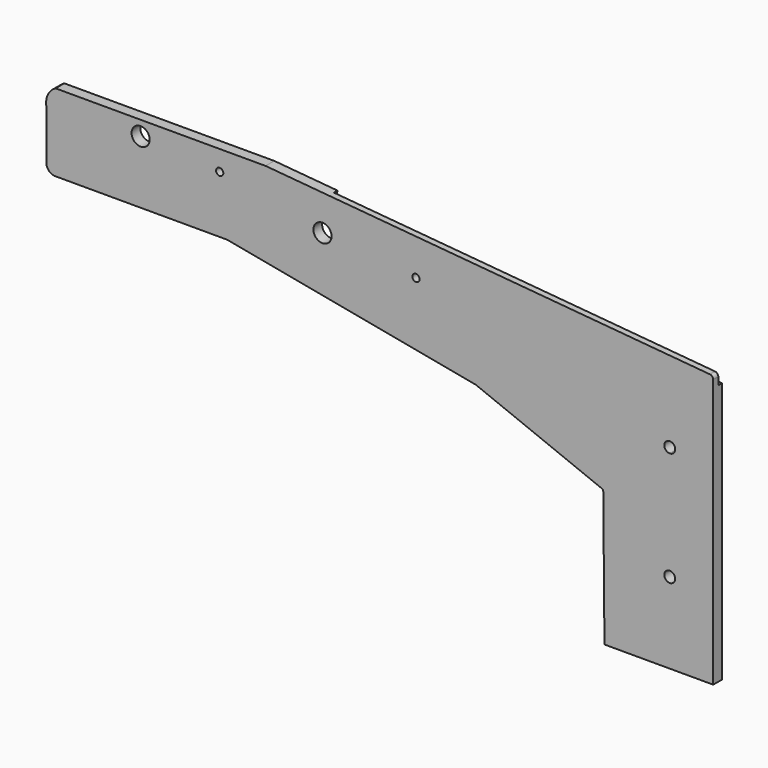
from build123d import *

# Parameters (mm, degrees)
F0_R      = 2
F1_DEPTH  = 6
F3_DEPTH  = 6.001
F5_DEPTH  = 6.001
F6_R      = 5
F7_DEPTH  = 6.001
F8_DEPTH  = 585
F9_R      = 2
F10_DEPTH = 6.001
F12_DEPTH = 2.5
F13_R     = 2


# Not quite as in the source:
# - an extrude ends at something that could not be found from the text; its depth is read off the source's solid


with BuildPart() as f1:
    # F0 (on Front) → F1 (new body)
    with BuildSketch(Plane.XZ):
        with BuildLine():
            Line((61.1081310213, 8.0650188029), (-54.7722764313, 8.0650188029))
            ThreePointArc((-54.7722764313, 8.0650188029), (-58.9525619371, 3.7295520634), (-59.8848706484, -2.2203940898))
            Line((-59.8848706484, -2.2203940898), (-59.8848706484, -29.6689261496))
            ThreePointArc((-59.8848706484, -29.6689261496), (-58.4204045543, -33.2044600555), (-54.8848706484, -34.6689261496))
            Line((-54.8848706484, -34.6689261496), (-38.6363018323, -34.6689261496))
            Line((-38.6363018323, -34.6689261496), (39.8797094822, -34.6689261496))
            Line((39.8797094822, -34.6689261496), (177.1196573973, -60.5151057243))
            Line((177.1196573973, -60.5151057243), (247.381187493, -88.5924363301))
            Line((247.381187493, -88.5924363301), (248.0585300922, -163.5853774846))
            Line((248.0585300922, -163.5853774846), (308.0585300922, -163.5853774846))
            Line((308.0585300922, -163.5853774846), (308.0585300922, -13.5853774846))
            Line((308.0585300922, -13.5853774846), (61.1081310213, 8.0650188029))
        make_face()
        with Locations((35.7915443742, -3.0683759738)):
            Circle(F0_R, mode=Mode.SUBTRACT)
    extrude(amount=F1_DEPTH)

    # F2 (on face) → F3 (cut, through all)
    with BuildSketch(Plane.XZ.offset(6)):
        with BuildLine():
            ThreePointArc((92.5020176823, -9.2679053605), (88.9664837764, -17.8034392664), (97.5020176823, -14.2679053605))
            ThreePointArc((97.5020176823, -14.2679053605), (96.0375515883, -10.7323714546), (92.5020176823, -9.2679053605))
        make_face()
    extrude(amount=-F3_DEPTH, mode=Mode.SUBTRACT)

    # F4 (on face) → F5 (cut, through all)
    with BuildSketch(Plane.XZ.offset(6)):
        with BuildLine():
            ThreePointArc((284.0794362254, -115.9942394993), (281.9581158818, -121.1155598429), (287.0794362254, -118.9942394993))
            ThreePointArc((287.0794362254, -118.9942394993), (286.2007565689, -116.8729191558), (284.0794362254, -115.9942394993))
        make_face()
        with BuildLine():
            ThreePointArc((287.0794362254, -56.0820794532), (281.9581158818, -53.9607591097), (284.0794362254, -59.0820794532))
            ThreePointArc((284.0794362254, -59.0820794532), (286.2007565689, -58.2033997968), (287.0794362254, -56.0820794532))
        make_face()
    extrude(amount=-F5_DEPTH, mode=Mode.SUBTRACT)

    # F6 (on face) → F7 (cut, through all)
    with BuildSketch(Plane(origin=(0, 0, 0), x_dir=(-1, 0, 0), z_dir=(0, 1, 0))):
        with Locations((7.8367077125, 0)):
            Circle(F6_R)
    extrude(amount=-F7_DEPTH, mode=Mode.SUBTRACT)

    # F0 (on Front) → F8 (cut, through all)
    with BuildSketch(Plane.XZ):
        with BuildLine():
            Line((61.1081310213, 8.0650188029), (-54.7722764313, 8.0650188029))
            ThreePointArc((-54.7722764313, 8.0650188029), (-58.9525619371, 3.7295520634), (-59.8848706484, -2.2203940898))
            Line((-59.8848706484, -2.2203940898), (-59.8848706484, -29.6689261496))
            ThreePointArc((-59.8848706484, -29.6689261496), (-58.4204045543, -33.2044600555), (-54.8848706484, -34.6689261496))
            Line((-54.8848706484, -34.6689261496), (-38.6363018323, -34.6689261496))
            Line((-38.6363018323, -34.6689261496), (39.8797094822, -34.6689261496))
            Line((39.8797094822, -34.6689261496), (177.1196573973, -60.5151057243))
            Line((177.1196573973, -60.5151057243), (247.381187493, -88.5924363301))
            Line((247.381187493, -88.5924363301), (248.0585300922, -163.5853774846))
            Line((248.0585300922, -163.5853774846), (308.0585300922, -163.5853774846))
            Line((308.0585300922, -163.5853774846), (308.0585300922, -13.5853774846))
            Line((308.0585300922, -13.5853774846), (61.1081310213, 8.0650188029))
        make_face()
        with Locations((35.7915443742, -3.0683759738)):
            Circle(F0_R, mode=Mode.SUBTRACT)
    extrude(amount=-F8_DEPTH, mode=Mode.SUBTRACT)

    # F9 (on face) → F10 (cut, through all)
    with BuildSketch(Plane.XZ.offset(6)):
        with Locations((144.0575271969, -19.352506299)):
            Circle(F9_R)
    extrude(amount=-F10_DEPTH, mode=Mode.SUBTRACT)

    # F11 (on face) → F12 (cut)
    with BuildSketch(Plane(origin=(0, 0, 0), x_dir=(-1, 0, 0), z_dir=(0, 1, 0))):
        Polygon((-95.3768665934, -0.9623710934), (-95.9008827898, 5.0147023565), (-298.1252011792, -12.7145122896), (-308.0585300922, -13.5853774846), (-308.0585300922, -19.6083919751), (-297.6011849827, -18.6915857396), align=None)
    extrude(amount=-F12_DEPTH, mode=Mode.SUBTRACT)

    # F13
    f13_edges = [f1.edges().sort_by_distance(p)[0] for p in [
        (308.05853, -4.25, -13.585377),
    ]]
    fillet(f13_edges, radius=F13_R)


solid = f1.part
